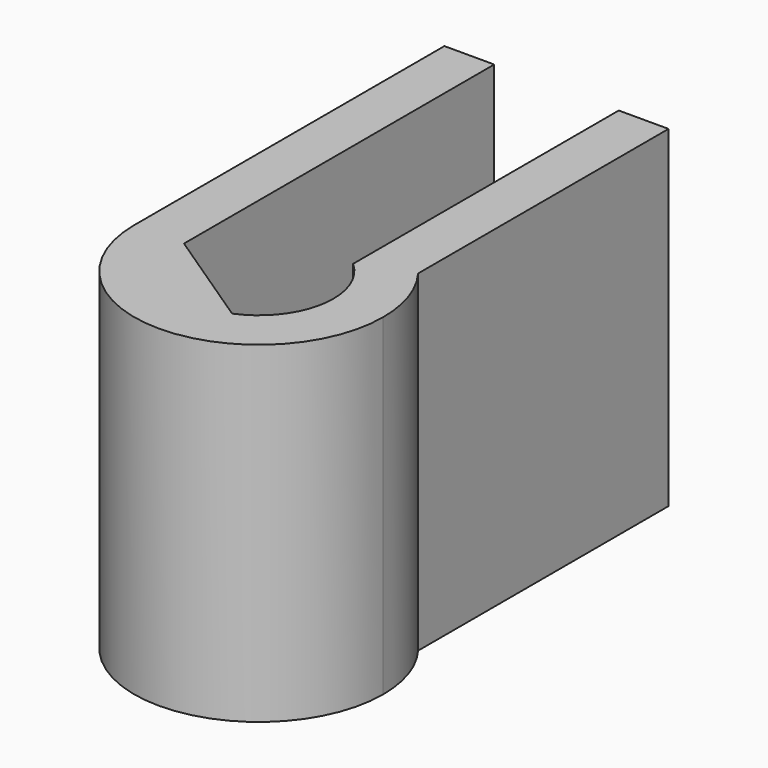
from build123d import *

# Parameters (mm, degrees)
F1_DEPTH = 10


# Not quite as in the source:
# - a feature names something its author has since deleted; it is built from what else it names


with BuildPart() as f1:
    # F0 (on Top) → F1 (new body)
    with BuildSketch(Plane.XY):
        with BuildLine():
            ThreePointArc((-3.75, 0), (-3.3541019662, 1.6770509831), (-2.25, 3))
            Line((-2.25, 3), (-2.25, 11.6770509831))
            Line((-2.25, 11.6770509831), (-3.75, 11.6770509831))
            Line((-3.75, 11.6770509831), (-3.75, 0))
        make_face()
        with BuildLine():
            ThreePointArc((1.5, 1.6770509831), (2.0539595906, 0.9185586535), (2.25, 0))
            ThreePointArc((2.25, 0), (1.8708286934, -1.25), (0.8611111111, -2.0786985482))
            ThreePointArc((0.8611111111, -2.0786985482), (-1.25, -1.8708286934), (-2.25, 0))
            Line((-2.25, 0), (-2.25, 3))
            ThreePointArc((-2.25, 3), (-3.3541019662, 1.6770509831), (-3.75, 0))
            ThreePointArc((-3.75, 0), (0, -3.75), (3.75, 0))
            ThreePointArc((3.75, 0), (3.5575623677, 1.1858541226), (3, 2.25))
            ThreePointArc((3, 2.25), (2.3269511721, 2.9407139002), (1.5, 3.4369317712))
            Line((1.5, 3.4369317712), (1.5, 1.6770509831))
        make_face()
        with BuildLine():
            Line((1.5, 11.6770509831), (1.5, 3.4369317712))
            ThreePointArc((1.5, 3.4369317712), (2.3269511721, 2.9407139002), (3, 2.25))
            Line((3, 2.25), (3, 11.6770509831))
            Line((3, 11.6770509831), (1.5, 11.6770509831))
        make_face()
        with BuildLine():
            ThreePointArc((-2.25, 0), (-1.25, -1.8708286934), (0.8611111111, -2.0786985482))
            Line((0.8611111111, -2.0786985482), (-2.25, 0))
        make_face()
    extrude(amount=F1_DEPTH)


solid = f1.part
